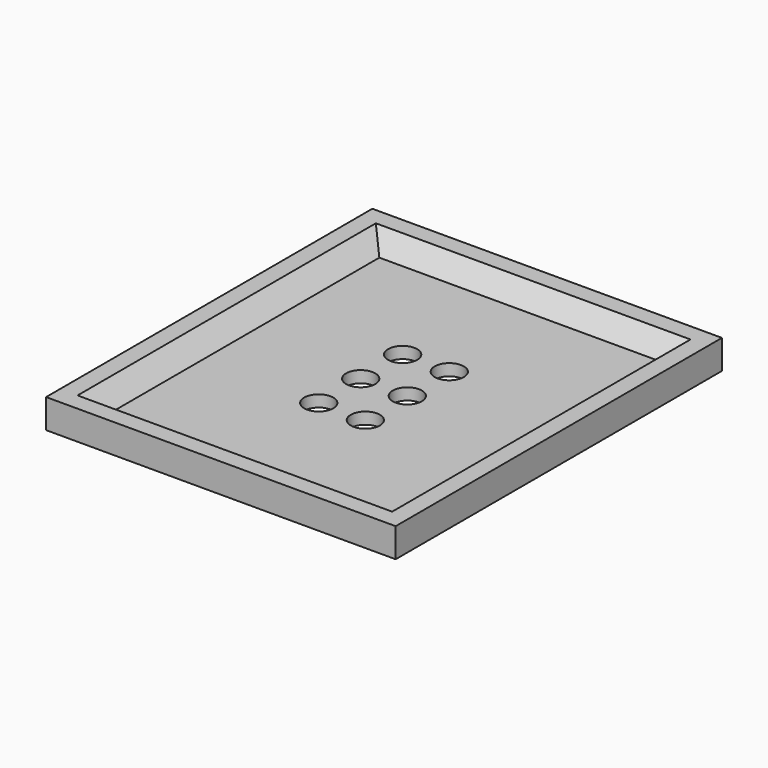
from build123d import *

# Parameters (mm, degrees)
F0_W         = 88.9
F0_H         = 6.35
F1_DEPTH     = 76.2
F2_T         = -2.54
F3_T4_DEPTH  = 83.82
F3_T9_DEPTH  = 71.12
F3_T14_DEPTH = 83.82
F3_T19_DEPTH = 71.12
F5_D         = 6.35
F5_DEPTH     = 12.7
F5_TIP       = 1.9077324654


# Not quite as in the source:
# - a fillet or chamfer that OpenCascade refuses, or shapes differently, is made with other operations: its cross-section is extruded or revolved along the edge and cut away or added


with BuildPart() as f1:
    # F0 (on Right) → F1 (new body)
    with BuildSketch(Plane.YZ):
        with Locations((12.1882097632, -0.3118954591)):
            Rectangle(F0_W, F0_H)
    extrude(amount=F1_DEPTH)

    # F2
    f2_openings = [f1.faces().sort_by_distance(p)[0] for p in [
        (38.1, 12.18821, 2.863105),
    ]]
    offset(amount=F2_T, openings=f2_openings)

    # F3: chamfer of 5.08 on 4 edges, made by hand


with BuildPart() as f3_tool2:
    # F3_s3 → F3_t4 (new body)
    with BuildSketch(Plane.XZ.offset(-54.0982097632)):
        Polygon((2.54, 4.1331045409), (7.62, -0.9468954591), (2.54, -0.9468954591), align=None)
    extrude(amount=F3_T4_DEPTH)

    split(bisect_by=Plane.XY.offset(2.8631045409), keep=Keep.BOTTOM)


with BuildPart() as f1_1:
    add(f1.part)

    # F3_t1: union F3_tool2
    add(f3_tool2.part)


with BuildPart() as f3_tool7:
    # F3_s8 → F3_t9 (new body)
    with BuildSketch(Plane.YZ.offset(2.54)):
        Polygon((-29.7217902368, 4.1331045409), (-24.6417902368, -0.9468954591), (-29.7217902368, -0.9468954591), align=None)
    extrude(amount=F3_T9_DEPTH)

    split(bisect_by=Plane.XY.offset(2.8631045409), keep=Keep.BOTTOM)


with BuildPart() as f1_2:
    add(f1_1.part)

    # F3_t6: union F3_tool7
    add(f3_tool7.part)


with BuildPart() as f3_tool12:
    # F3_s13 → F3_t14 (new body)
    with BuildSketch(Plane.XZ.offset(-54.0982097632)):
        Polygon((73.66, 4.1331045409), (68.58, -0.9468954591), (73.66, -0.9468954591), align=None)
    extrude(amount=F3_T14_DEPTH)

    split(bisect_by=Plane.XY.offset(2.8631045409), keep=Keep.BOTTOM)


with BuildPart() as f1_3:
    add(f1_2.part)

    # F3_t11: union F3_tool12
    add(f3_tool12.part)


with BuildPart() as f3_tool17:
    # F3_s18 → F3_t19 (new body)
    with BuildSketch(Plane.YZ.offset(73.66)):
        Polygon((54.0982097632, 4.1331045409), (49.0182097632, -0.9468954591), (54.0982097632, -0.9468954591), align=None)
    extrude(amount=-F3_T19_DEPTH)

    split(bisect_by=Plane.XY.offset(2.8631045409), keep=Keep.BOTTOM)


with BuildPart() as f1_4:
    add(f1_3.part)

    # F3_t16: union F3_tool17
    add(f3_tool17.part)

    # F5
    with Locations(Plane.XY.offset(-0.9468954591)):
        with Locations((33.02, 23.6182097632), (43.18, 23.6182097632), (43.18, 12.1882097632), (33.02, 12.1882097632), (33.02, 0.7582097632), (43.18, 0.7582097632)):
            Hole(F5_D / 2, depth=F5_DEPTH)
            with Locations((0, 0, -(F5_DEPTH + F5_TIP / 2))):  # 118° drill point
                Cone(0, F5_D / 2, F5_TIP, mode=Mode.SUBTRACT)


solid = f1_4.part
